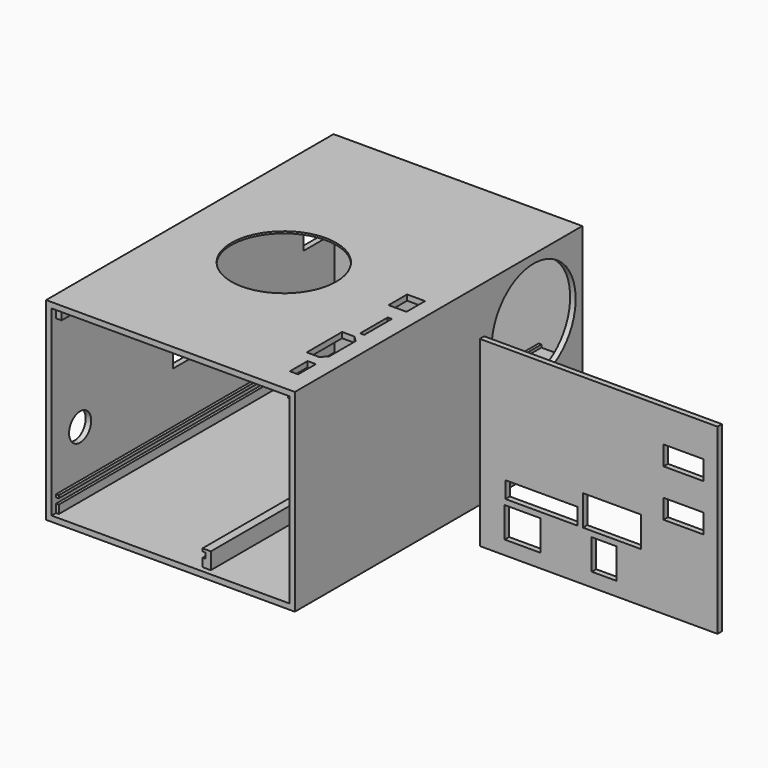
from build123d import *

# Parameters (mm, degrees)
F0_W      = 90
F0_H      = 130
F1_DEPTH  = 70
F2_T      = -2
F3_W      = 4
F3_H      = 2
F3_W_2    = 6
F4_DEPTH  = 6
F5_W      = 1
F5_H      = 3
F5_H_2    = 1
F6_DEPTH  = 103
F7_W      = 2
F7_H      = 3.7837837838
F8_DEPTH  = 5
F10_DEPTH = 70
F11_W     = 6.5
F11_H     = 8.4
F11_W_2   = 1.5
F11_H_2   = 12.5
F11_W_3   = 3
F11_H_3   = 8
F11_R     = 19
F12_DEPTH = 2
F11_R_2   = 32
F13_DEPTH = 1.3
F11_W_4   = 2
F11_H_4   = 6
F14_DEPTH = 2
F15_W     = 1
F15_H     = 1
F16_DEPTH = 40
F17_R     = 19
F18_DEPTH = 2
F19_W     = 86
F19_H     = 66
F19_W_2   = 13
F19_H_2   = 11
F19_W_3   = 26
F19_H_3   = 6
F19_W_4   = 9
F19_W_5   = 21
F19_W_6   = 14.5
F19_H_4   = 7
F20_DEPTH = 2
F21_W     = 3
F21_H     = 7
F22_DEPTH = 2
F23_W     = 14
F23_H     = 27
F23_H_2   = 17
F23_R     = 5
F24_DEPTH = 2
F23_W_2   = 4
F23_H_3   = 4
F25_DEPTH = 4


# Not quite as in the source:
# - a feature names something its author has since deleted; it is built from what else it names


with BuildPart() as f1:
    # F0 (on Top) → F1 (new body)
    with BuildSketch(Plane.XY):
        with Locations((10.2467668056, 1.9931593537)):
            Rectangle(F0_W, F0_H)
    extrude(amount=F1_DEPTH)

    # F2
    f2_openings = [f1.faces().sort_by_distance(p)[0] for p in [
        (10.246767, -63.006841, 35),
    ]]
    offset(amount=F2_T, openings=f2_openings)

    # F3 (on face) → F4 (join)
    with BuildSketch(Plane.XY.offset(2)):
        with Locations((-30.7532331944, 42.9931593537)):
            Rectangle(F3_W, F3_H)
        with Locations((20.2467668056, 42.9931593537)):
            Rectangle(F3_W_2, F3_H)
    extrude(amount=F4_DEPTH)

    # F5 (on face) → F6 (join)
    with BuildSketch(Plane.XZ.offset(-41.9931593537)):
        Polygon((20.2467668056, 7), (21.2467668056, 7), (21.2467668056, 5), (20.2467668056, 5), (20.2467668056, 2), (23.2467668056, 2), (23.2467668056, 8), (20.2467668056, 8), align=None)
        with Locations((-32.2532331944, 3.5)):
            Rectangle(F5_W, F5_H)
        with Locations((-32.2532331944, 7.5)):
            Rectangle(F5_W, F5_H_2)
    extrude(amount=F6_DEPTH)

    # F7 (on face) → F8 (join)
    with BuildSketch(Plane(origin=(53.2467668056, 0, 0), x_dir=(0, -1, 0), z_dir=(-1, 0, 0))):
        Polygon((-8.9931593537, 20.8918918919), (-8.9931593537, 17.1081081081), (-6.9931593537, 17.1081081081), (-6.9931593537, 19), (-6.9931593537, 20.8918918919), align=None)
        with Locations((48.0068406463, 19)):
            Rectangle(F7_W, F7_H)
    extrude(amount=F8_DEPTH)

    # F9 (on face) → F10 (cut)
    with BuildSketch(Plane.XZ.offset(49.0068406463)):
        Polygon((51.2467668056, 20.1351351351), (53.2467668056, 20.8918918919), (48.2467668056, 20.8918918919), (48.2467668056, 19), (49.2467668056, 19.3783783784), (49.2467668056, 18.8918918919), (51.2467668056, 18.8918918919), align=None)
        Polygon((48.2467668056, 17.1081081081), (53.2467668056, 17.1081081081), (48.2467668056, 18), align=None)
    extrude(amount=-F10_DEPTH, mode=Mode.SUBTRACT)

    # F11 (on face) → F12 (cut)
    with BuildSketch(Plane(origin=(0, 0, 68), x_dir=(1, 0, 0), z_dir=(0, 0, -1))):
        with Locations((45.9967668056, 0.8068406463)):
            Rectangle(F11_W, F11_H)
        with Locations((47.9967668056, 17.2568406463)):
            Rectangle(F11_W_2, F11_H_2)
        Polygon((49.2467668056, 28.0068406463), (49.2467668056, 40.0068406463), (47.2467668056, 42.0068406463), (42.7467668056, 42.0068406463), (42.7467668056, 26.0068406463), (47.2467668056, 26.0068406463), align=None)
        with Locations((47.7467668056, 50.0068406463)):
            Rectangle(F11_W_3, F11_H_3)
        with Locations((3.2467668056, 3.0068406463)):
            Circle(F11_R)
    extrude(amount=-F12_DEPTH, mode=Mode.SUBTRACT)

    # F11 (on face) → F13 (cut)
    with BuildSketch(Plane(origin=(0, 0, 68), x_dir=(1, 0, 0), z_dir=(0, 0, -1))):
        with Locations((3.2467668056, 3.0068406463)):
            Circle(F11_R_2)
        with Locations((3.2467668056, 3.0068406463)):
            Circle(F11_R, mode=Mode.SUBTRACT)
    extrude(amount=-F13_DEPTH, mode=Mode.SUBTRACT)

    # F11 (on face) → F14 (join)
    with BuildSketch(Plane(origin=(0, 0, 68), x_dir=(1, 0, 0), z_dir=(0, 0, -1))):
        with Locations((52.2467668056, -5.9931593537)):
            Rectangle(F11_W_4, F11_H_4)
        with Locations((52.2467668056, 57.0068406463)):
            Rectangle(F11_W_4, F11_H_3)
    extrude(amount=F14_DEPTH)

    # F15 (on face) → F16 (join)
    with BuildSketch(Plane.XZ.offset(-64.9931593537)):
        Polygon((53.2467668056, 26.8), (53.2467668056, 27.8), (42.0467668056, 27.8), (42.0467668056, 28.8), (41.0467668056, 28.8), (41.0467668056, 26.8), align=None)
        with Locations((41.5467668056, 67.5)):
            Rectangle(F15_W, F15_H)
    extrude(amount=F16_DEPTH)

    # F17 (on face) → F18 (cut)
    with BuildSketch(Plane(origin=(53.2467668056, 0, 0), x_dir=(0, -1, 0), z_dir=(-1, 0, 0))):
        with Locations((-44.9931593537, 48)):
            Circle(F17_R)
    extrude(amount=-F18_DEPTH, mode=Mode.SUBTRACT)

    # F21 (on face) → F22 (cut)
    with BuildSketch(Plane(origin=(53.2467668056, 0, 0), x_dir=(0, -1, 0), z_dir=(-1, 0, 0))):
        with Locations((-63.4931593537, 5.5)):
            Rectangle(F21_W, F21_H)
    extrude(amount=-F22_DEPTH, mode=Mode.SUBTRACT)

    # F23 (on face) → F24 (cut)
    with BuildSketch(Plane(origin=(-34.7532331944, 0, 0), x_dir=(0, -1, 0), z_dir=(-1, 0, 0))):
        with Locations((-57.9931593537, 53.5)):
            Rectangle(F23_W, F23_H)
        with Locations((1.0068406463, 35)):
            Rectangle(F23_W, F23_H_2)
        with Locations((50.1068407744, 25)):
            Circle(F23_R)
    extrude(amount=-F24_DEPTH, mode=Mode.SUBTRACT)

    # F23 (on face) → F25 (join)
    with BuildSketch(Plane(origin=(-34.7532331944, 0, 0), x_dir=(0, -1, 0), z_dir=(-1, 0, 0))):
        with Locations((59.0068406463, 66)):
            Rectangle(F23_W_2, F23_H_3)
    extrude(amount=-F25_DEPTH)


with BuildPart() as f20:
    # F19 (on Front) → F20 (new body)
    with BuildSketch(Plane.XZ):
        with Locations((116.3490213752, 35)):
            Rectangle(F19_W, F19_H)
        with Locations((88.8490213752, 12.5)):
            Rectangle(F19_W_2, F19_H_2, mode=Mode.SUBTRACT)
        with Locations((95.6490213752, 23)):
            Rectangle(F19_W_3, F19_H_3, mode=Mode.SUBTRACT)
        with Locations((118.3490213752, 12.5)):
            Rectangle(F19_W_4, F19_H_2, mode=Mode.SUBTRACT)
        with Locations((121.1490213752, 25.5)):
            Rectangle(F19_W_5, F19_H_2, mode=Mode.SUBTRACT)
        with Locations((147.0990213752, 35.5)):
            Rectangle(F19_W_6, F19_H_4, mode=Mode.SUBTRACT)
        with Locations((147.0990213752, 52.5)):
            Rectangle(F19_W_6, F19_H_4, mode=Mode.SUBTRACT)
    extrude(amount=F20_DEPTH)


solid = Compound([f1.part, f20.part])
